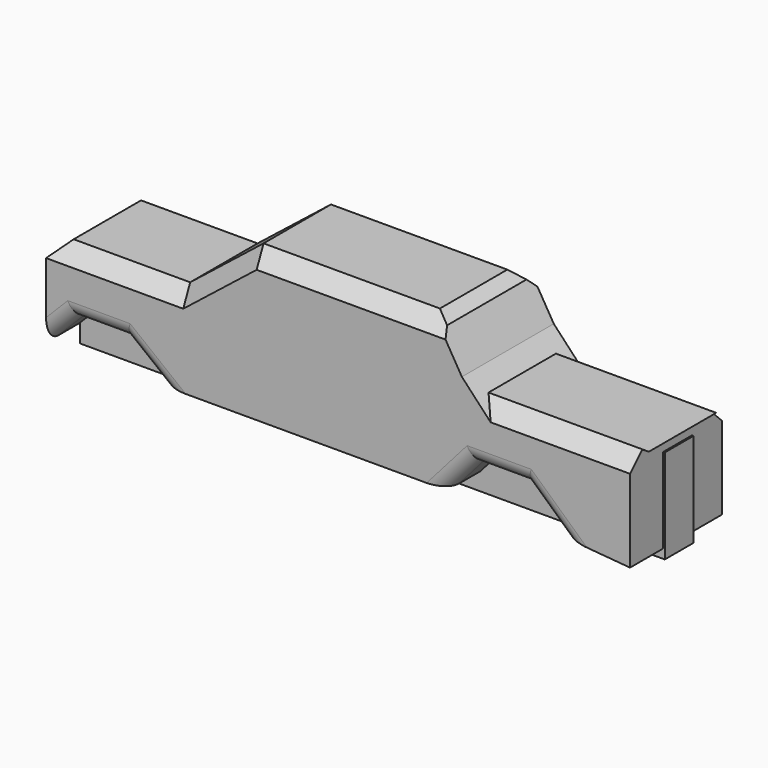
from build123d import *

# Parameters (mm, degrees)
F1_DEPTH      = 38.1
F2_T1_DEPTH   = 64.2282991577
F2_T3_DEPTH   = 53.4259096179
F2_T8_DEPTH   = 69.8505852304
F2_T13_DEPTH  = 69.8505852304
F2_T18_DEPTH  = 57.18488627
F2_T23_DEPTH  = 57.18488627
F2_T29_DEPTH  = 57.18488627
F2_T33_DEPTH  = 56.7864356516
F2_T40_DEPTH  = 56.7864356516
F2_T44_DEPTH  = 57.18488627
F3_R          = 5.5188922036
F4_R          = 5.08
F5_SIZE       = 5.08
F6_SIZE       = 5.08
F8_DEPTH      = 5.842
F8_DEPTH_BACK = 25.4


# Not quite as in the source:
# - a fillet or chamfer that OpenCascade refuses, or shapes differently, is made with other operations: its cross-section is extruded or revolved along the edge and cut away or added


with BuildPart() as f1:
    # F0 (on Front) → F1 (new body)
    with BuildSketch(Plane.XZ):
        Polygon((68.3197870099, -30.5711814668), (90.9013386944, -32.4848717284), (90.9013386944, -19.5518693537), (90.9013386944, -0.0529484335), (93.0701802755, 0), (60.7909710004, 0), (39.9160396704, 0), (35.1392942637, 5.0951969111), (26.685241969, 19.2868879506), (6.6764656577, 19.2868879506), (-19.6780025163, 19.2868879506), (-34.6921224135, 19.2868879506), (-59.0340113345, 0), (-76.2522614858, 0), (-85.7398739654, 0), (-102.7562974073, 0), (-102.7562974073, -29.6926991102), (-93.4295707114, -20.2366987188), (-86.7940447176, -20.2366987188), (-78.7120151127, -20.2366987188), (-76.6338963938, -20.2366987188), (-64.6562974073, -29.6926991102), (-40.7615778127, -29.6926991102), (-19.6780025163, -29.6926991102), (0, -29.6926991102), (14.0557177055, -29.6926991102), (30.2197870099, -29.6926991102), (39.1803090661, -19.5023065498), (56.2228657745, -19.5023065498), align=None)
    extrude(amount=F1_DEPTH)

    # F2: chamfer of 5.08 on 6 edges, made by hand

    # F2_s2 → F2_t1 (cut)
    with BuildSketch(Plane.XZ.offset(-13.0641495789)):
        Polygon((-102.7562974073, -5.08), (-97.6762974073, 0), (-102.7562974073, 0), align=None)
    extrude(amount=F2_T1_DEPTH, mode=Mode.SUBTRACT)

    # F2_s4 → F2_t3 (cut)
    with BuildSketch(Plane.XZ.offset(-7.6629548089)):
        Polygon((23.7983706465, 19.2868879506), (28.1626838525, 16.8067283763), (26.685241969, 19.2868879506), align=None)
    extrude(amount=F2_T3_DEPTH, mode=Mode.SUBTRACT)


with BuildPart() as f2_tool6:
    # F2_s7 → F2_t8 (new body)
    with BuildSketch(Plane.YZ.offset(-115.8204469861)):
        Polygon((-38.1, -5.08), (-33.02, 0), (-38.1, 0), align=None)
    extrude(amount=F2_T8_DEPTH)

    split(bisect_by=Plane(origin=(-22.7676995967, 0, 28.7350046307), x_dir=(0, 1, 0), z_dir=(-0.6210240643, 0, 0.7837914975)), keep=Keep.TOP)


with BuildPart() as f1_1:
    add(f1.part)

    # F2_t5: cut F2_tool6
    add(f2_tool6.part, mode=Mode.SUBTRACT)


with BuildPart() as f2_tool11:
    # F2_s12 → F2_t13 (new body)
    with BuildSketch(Plane.YZ.offset(-45.9698617557)):
        Polygon((-5.08, 0), (0, -5.08), (0, 0), align=None)
    extrude(amount=-F2_T13_DEPTH)

    split(bisect_by=Plane(origin=(-22.7676995967, 0, 28.7350046307), x_dir=(0, 1, 0), z_dir=(-0.6210240643, 0, 0.7837914975)), keep=Keep.TOP)


with BuildPart() as f1_2:
    add(f1_1.part)

    # F2_t10: cut F2_tool11
    add(f2_tool11.part, mode=Mode.SUBTRACT)


with BuildPart() as f2_tool16:
    # F2_s17 → F2_t18 (new body)
    with BuildSketch(Plane(origin=(-1.6848534543, 0, -1.3349654126), x_dir=(0, 1, 0), z_dir=(-0.7837914975, 0, -0.6210240643))):
        Polygon((-38.1, -31.5815416486), (-33.02, -36.6615416486), (-38.1, -36.6615416486), align=None)
    extrude(amount=F2_T18_DEPTH)

    split(bisect_by=Plane.XY, keep=Keep.TOP)


with BuildPart() as f1_3:
    add(f1_2.part)

    # F2_t15: cut F2_tool16
    add(f2_tool16.part, mode=Mode.SUBTRACT)


with BuildPart() as f2_tool21:
    # F2_s22 → F2_t23 (new body)
    with BuildSketch(Plane(origin=(-1.6848534543, 0, -1.3349654126), x_dir=(0, 1, 0), z_dir=(-0.7837914975, 0, -0.6210240643))):
        Polygon((-5.08, -36.6615416486), (0, -31.5815416486), (0, -36.6615416486), align=None)
    extrude(amount=F2_T23_DEPTH)

    split(bisect_by=Plane.XY, keep=Keep.TOP)


with BuildPart() as f1_4:
    add(f1_3.part)

    # F2_t20: cut F2_tool21
    add(f2_tool21.part, mode=Mode.SUBTRACT)


with BuildPart() as f2_tool27:
    # F2_s28 → F2_t29 (new body)
    with BuildSketch(Plane(origin=(-1.6848534543, 0, -1.3349654126), x_dir=(0, 1, 0), z_dir=(-0.7837914975, 0, -0.6210240643))):
        Polygon((-38.1, -31.5815416486), (-33.02, -36.6615416486), (-38.1, -36.6615416486), align=None)
    extrude(amount=F2_T29_DEPTH)

    split(bisect_by=Plane.XY, keep=Keep.BOTTOM)


with BuildPart() as f2_tool31:
    # F2_s32 → F2_t33 (new body)
    with BuildSketch(Plane.YZ.offset(-102.7562974073)):
        Polygon((-38.1, -5.08), (-33.02, 0), (-38.1, 0), align=None)
    extrude(amount=F2_T33_DEPTH)

    split(bisect_by=Plane(origin=(-22.7676995967, 0, 28.7350046307), x_dir=(0, 1, 0), z_dir=(0.6210240643, 0, -0.7837914975)), keep=Keep.TOP)


with BuildPart() as f2_tool27_1:
    add(f2_tool27.part)

    # F2_t35: intersect F2_tool31
    add(f2_tool31.part, mode=Mode.INTERSECT)


with BuildPart() as f1_5:
    add(f1_4.part)

    # F2_t25: cut F2_tool27
    add(f2_tool27_1.part, mode=Mode.SUBTRACT)


with BuildPart() as f2_tool38:
    # F2_s39 → F2_t40 (new body)
    with BuildSketch(Plane.YZ.offset(-45.9698617557)):
        Polygon((-5.08, 0), (0, -5.08), (0, 0), align=None)
    extrude(amount=-F2_T40_DEPTH)

    split(bisect_by=Plane(origin=(-22.7676995967, 0, 28.7350046307), x_dir=(0, 1, 0), z_dir=(0.6210240643, 0, -0.7837914975)), keep=Keep.TOP)


with BuildPart() as f2_tool42:
    # F2_s43 → F2_t44 (new body)
    with BuildSketch(Plane(origin=(-1.6848534543, 0, -1.3349654126), x_dir=(0, 1, 0), z_dir=(-0.7837914975, 0, -0.6210240643))):
        Polygon((-5.08, -36.6615416486), (0, -31.5815416486), (0, -36.6615416486), align=None)
    extrude(amount=F2_T44_DEPTH)

    split(bisect_by=Plane.XY, keep=Keep.BOTTOM)


with BuildPart() as f2_tool38_1:
    add(f2_tool38.part)

    # F2_t46: intersect F2_tool42
    add(f2_tool42.part, mode=Mode.INTERSECT)


with BuildPart() as f1_6:
    add(f1_5.part)

    # F2_t36: cut F2_tool38
    add(f2_tool38_1.part, mode=Mode.SUBTRACT)

    # F3
    f3_edges = [f1_6.edges().sort_by_distance(p)[0] for p in [
        (62.271326, 0, -25.036744),
        (47.701587, 0, -19.502307),
        (34.700048, 0, -24.597503),
    ]]
    fillet(f3_edges, radius=F3_R)

    # F4
    f4_edges = [f1_6.edges().sort_by_distance(p)[0] for p in [
        (34.700048, -38.1, -24.597503),
        (47.701587, -38.1, -19.502307),
        (62.271326, -38.1, -25.036744),
        (-70.645097, 0, -24.964699),
        (-85.031734, 0, -20.236699),
        (-98.092934, 0, -24.964699),
        (-85.031734, -38.1, -20.236699),
        (-70.645097, -38.1, -24.964699),
        (-98.092934, -38.1, -24.964699),
    ]]
    fillet(f4_edges, radius=F4_R)

    # F5
    f5_edges = [f1_6.edges().sort_by_distance(p)[0] for p in [
        (66.49311, -38.1, 0),
        (66.49311, 0, 0),
    ]]
    chamfer(f5_edges, length=F5_SIZE)

    # F6
    f6_edges = [f1_6.edges().sort_by_distance(p)[0] for p in [
        (-1.356857, 0, 19.286888),
        (-1.356857, -38.1, 19.286888),
    ]]
    chamfer(f6_edges, length=F6_SIZE)

    # F7 (on face) → F8 (join, two sides)
    with BuildSketch(Plane(origin=(0, 0, -29.6926991102), x_dir=(1, 0, 0), z_dir=(0, 0, -1))) as f8_sk:
        Polygon((-102.5345399976, 24.3232287467), (-102.5345399976, 12.4534405768), (90.11746943, 12.4534405768), (91.410189867, 12.4534405768), (91.410189867, 24.3232287467), align=None)
    extrude(amount=F8_DEPTH)
    extrude(f8_sk.sketch, amount=-F8_DEPTH_BACK)


solid = f1_6.part
